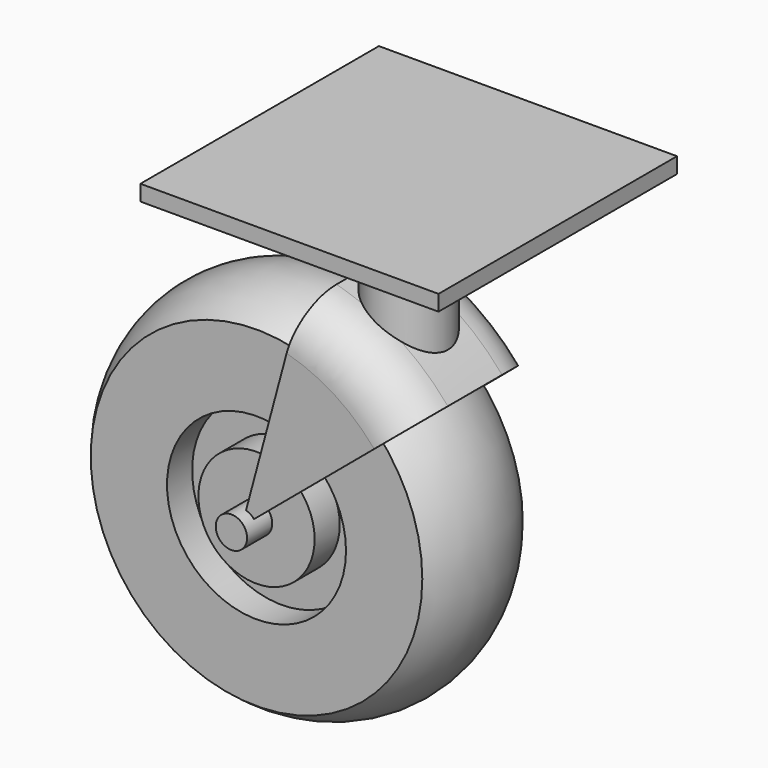
from build123d import *

# Parameters (mm, degrees)
F3_ANGLE_START = 40
F3_ANGLE       = 35
F6_R           = 7.9375
F5_W           = 60.325
F5_H           = 60.325
F8_DEPTH       = 3.175


with BuildPart() as f1:
    # F0 (on Top) → F1 (revolve)
    with BuildSketch(Plane.XY):
        with BuildLine():
            Line((3.175, -19.05), (3.175, -12.7))
            Line((3.175, -12.7), (11.7603466757, -12.7))
            Line((11.7603466757, -12.7), (11.7603466757, -6.35))
            Line((11.7603466757, -6.35), (18.1103466757, -6.35))
            Line((18.1103466757, -6.35), (18.1103466757, -12.7))
            Line((18.1103466757, -12.7), (33.5471935048, -12.7))
            ThreePointArc((33.5471935048, -12.7), (38.1, 0), (33.5471935048, 12.7))
            Line((33.5471935048, 12.7), (18.1103466757, 12.7))
            Line((18.1103466757, 12.7), (18.1103466757, 6.35))
            Line((18.1103466757, 6.35), (11.7603466757, 6.35))
            Line((11.7603466757, 6.35), (11.7603466757, 12.7))
            Line((11.7603466757, 12.7), (3.175, 12.7))
            Line((3.175, 12.7), (3.175, 19.05))
            Line((3.175, 19.05), (0, 19.05))
            Line((0, 19.05), (0, -19.05))
            Line((0, -19.05), (3.175, -19.05))
        make_face()
    revolve(axis=Axis((0, 0, 0), (0, -1, 0)))

    # F2 (on Top) → F3 (revolve)
    with BuildSketch(Plane.XY, mode=Mode.PRIVATE) as f3_sk:
        with BuildLine():
            Line((0, 16.383), (0, 13.208))
            Line((0, 13.208), (34.925, 13.208))
            ThreePointArc((34.925, 13.208), (39.4151280605, 11.3481280605), (41.275, 6.858))
            Line((41.275, 6.858), (41.275, 0))
            Line((41.275, 0), (41.275, -6.858))
            ThreePointArc((41.275, -6.858), (39.4151280605, -11.3481280605), (34.925, -13.208))
            Line((34.925, -13.208), (0, -13.208))
            Line((0, -13.208), (0, -16.383))
            Line((0, -16.383), (34.925, -16.383))
            ThreePointArc((34.925, -16.383), (41.6601920908, -13.5931920908), (44.45, -6.858))
            Line((44.45, -6.858), (44.45, 0))
            Line((44.45, 0), (44.45, 6.858))
            ThreePointArc((44.45, 6.858), (41.6601920908, 13.5931920908), (34.925, 16.383))
            Line((34.925, 16.383), (0, 16.383))
        make_face()
    revolve(f3_sk.sketch.rotate(Axis((0, 23.489471525, 0), (0, -1, 0)), F3_ANGLE_START), axis=Axis((0, 23.489471525, 0), (0, -1, 0)), revolution_arc=F3_ANGLE)

    # F6 (on offset) → F7 (join, up to the next surface of F1)
    with BuildSketch(Plane.XY.offset(63.5)):
        with Locations((20.6375, 0)):
            Circle(F6_R)
    extrude(until=Until.NEXT, dir=(0, 0, -1))

    # F5 (on offset) → F8 (join)
    with BuildSketch(Plane.XY.offset(63.5)):
        with Locations((20.6375, 0)):
            Rectangle(F5_W, F5_H)
    extrude(amount=-F8_DEPTH)


solid = f1.part
